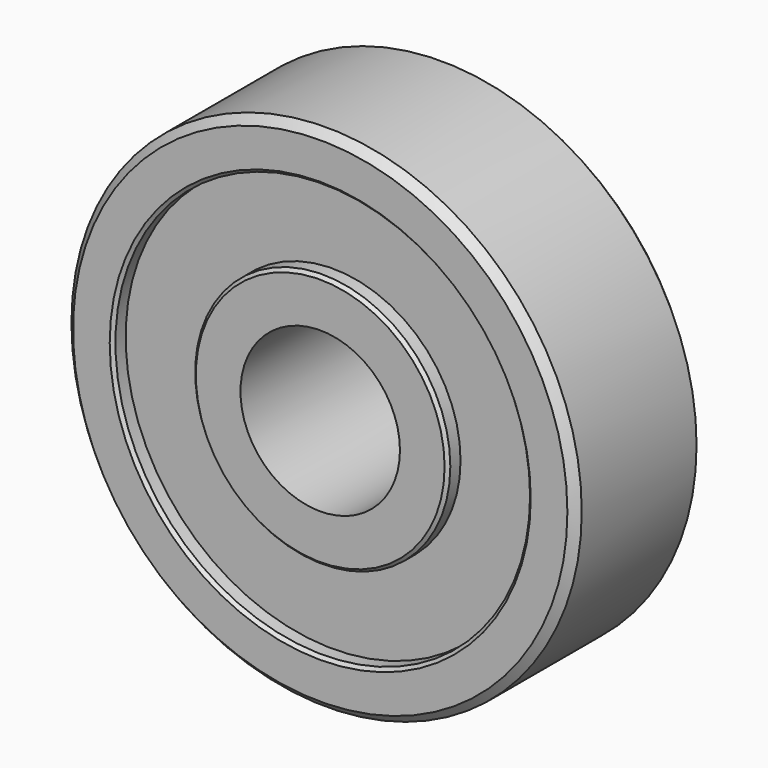
from build123d import *

# Parameters (mm, degrees)
F0_R     = 8
F0_R_2   = 2.5
F1_DEPTH = 2.5
F2_R     = 6.5
F2_R_2   = 4
F3_DEPTH = 0.5
F4_SIZE  = 0.25
F5_SIZE  = 0.1


# Not quite as in the source:
# - a pattern or mirror of a feature is missing from the dataset's text; its kind, count and spacing are read off the source's solid


with BuildPart() as f1:
    # F0 (on Front) → F1 (new body, symmetric)
    with BuildSketch(Plane.XZ):
        Circle(F0_R)
        Circle(F0_R_2, mode=Mode.SUBTRACT)
    extrude(amount=F1_DEPTH, both=True)

    # F2 (on face) → F3 (cut)
    with BuildSketch(Plane.XZ.offset(2.5)):
        Circle(F2_R)
        Circle(F2_R_2, mode=Mode.SUBTRACT)
    f3 = extrude(amount=-F3_DEPTH, mode=Mode.SUBTRACT)

    # F3_copies: F3 across plane
    add(f3.mirror(Plane.ZX), mode=Mode.SUBTRACT)

    # F4
    f4_edges = [f1.edges().sort_by_distance(p)[0] for p in [
        (-8, -2.5, 0),
        (-8, 2.5, 0),
    ]]
    chamfer(f4_edges, length=F4_SIZE)

    # F5
    f5_edges = [f1.edges().sort_by_distance(p)[0] for p in [
        (-6.5, -2.5, 0),
        (-4, -2.5, 0),
        (-6.5, 2.5, 0),
        (-4, 2.5, 0),
    ]]
    chamfer(f5_edges, length=F5_SIZE)


solid = f1.part
